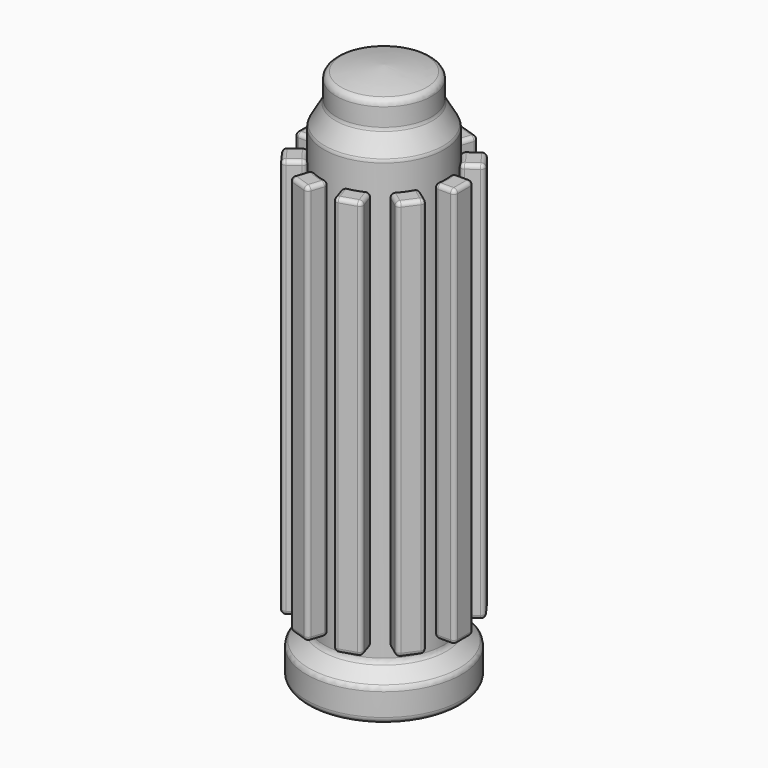
from build123d import *

# Parameters (mm, degrees)
F2_R     = 1.6
F4_W     = 6
F4_H     = 100
F6_R     = 1
F7_COUNT = 10


with BuildPart() as f1:
    # F0 (on Front) → F1 (revolve)
    with BuildSketch(Plane.XZ):
        with BuildLine():
            Line((0, 135), (0, 125))
            Line((0, 125), (10.75, 125))
            Line((10.75, 125), (10.75, 0))
            Line((10.75, 0), (19.325, 0))
            Line((19.325, 0), (19.325, 8))
            Line((19.325, 8), (15, 11.6291059048))
            Line((15, 11.6291059048), (15, 121.6291059048))
            Line((15, 121.6291059048), (11.8991128484, 127))
            Line((11.8991128484, 127), (11.8991128484, 133.2121827514))
            ThreePointArc((11.8991128484, 133.2121827514), (5.9891786333, 134.3698035294), (0, 135))
        make_face()
    revolve(axis=Axis((0, 0, 62.5), (0, 0, 1)))

    # F2
    f2_edges = [f1.edges().sort_by_distance(p)[0] for p in [
        (-11.899113, 0, 133.212183),
        (-11.899113, 0, 127),
        (-15, 0, 121.629106),
        (-15, 0, 11.629106),
        (-19.325, 0, 8),
        (-19.325, 0, 0),
    ]]
    fillet(f2_edges, radius=F2_R)


with BuildPart() as f5:
    # F4 (on offset) → F5 (new body, up to the next surface of F1)
    with BuildSketch(Plane.YZ.offset(20)):
        with Locations((0, 65)):
            Rectangle(F4_W, F4_H)
    extrude(until=Until.NEXT, target=f1.part, dir=(-1, 0, 0))

    # F6
    f6_edges = [f5.edges().sort_by_distance(p)[0] for p in [
        (20, -3, 65),
        (20, 3, 65),
        (20, 0, 115),
        (20, 0, 15),
        (17.348469, -3, 15),
        (17.348469, 3, 15),
        (17.348469, -3, 115),
        (17.348469, 3, 115),
        (14.696938, 3, 65),
        (14.924042, -1.507634, 115),
        (14.924042, 1.507634, 115),
        (14.696938, -3, 65),
        (14.924042, 1.507634, 15),
        (14.924042, -1.507634, 15),
    ]]
    fillet(f6_edges, radius=F6_R)


with BuildPart() as f7_1:
    # F7: instance of F5
    add(f5.part.rotate(Axis((0, 0, 62.5), (0, 0, 1)), 1 * 360 / F7_COUNT))


with BuildPart() as f7_2:
    # F7: instance of F5
    add(f5.part.rotate(Axis((0, 0, 62.5), (0, 0, 1)), 2 * 360 / F7_COUNT))


with BuildPart() as f7_3:
    # F7: instance of F5
    add(f5.part.rotate(Axis((0, 0, 62.5), (0, 0, 1)), 3 * 360 / F7_COUNT))


with BuildPart() as f7_4:
    # F7: instance of F5
    add(f5.part.rotate(Axis((0, 0, 62.5), (0, 0, 1)), 4 * 360 / F7_COUNT))


with BuildPart() as f7_5:
    # F7: instance of F5
    add(f5.part.rotate(Axis((0, 0, 62.5), (0, 0, 1)), 5 * 360 / F7_COUNT))


with BuildPart() as f7_6:
    # F7: instance of F5
    add(f5.part.rotate(Axis((0, 0, 62.5), (0, 0, 1)), 6 * 360 / F7_COUNT))


with BuildPart() as f7_7:
    # F7: instance of F5
    add(f5.part.rotate(Axis((0, 0, 62.5), (0, 0, 1)), 7 * 360 / F7_COUNT))


with BuildPart() as f7_8:
    # F7: instance of F5
    add(f5.part.rotate(Axis((0, 0, 62.5), (0, 0, 1)), 8 * 360 / F7_COUNT))


with BuildPart() as f7_9:
    # F7: instance of F5
    add(f5.part.rotate(Axis((0, 0, 62.5), (0, 0, 1)), 9 * 360 / F7_COUNT))


solid = Compound([f1.part, f5.part, f7_1.part, f7_2.part, f7_3.part, f7_4.part, f7_5.part, f7_6.part, f7_7.part, f7_8.part, f7_9.part])
